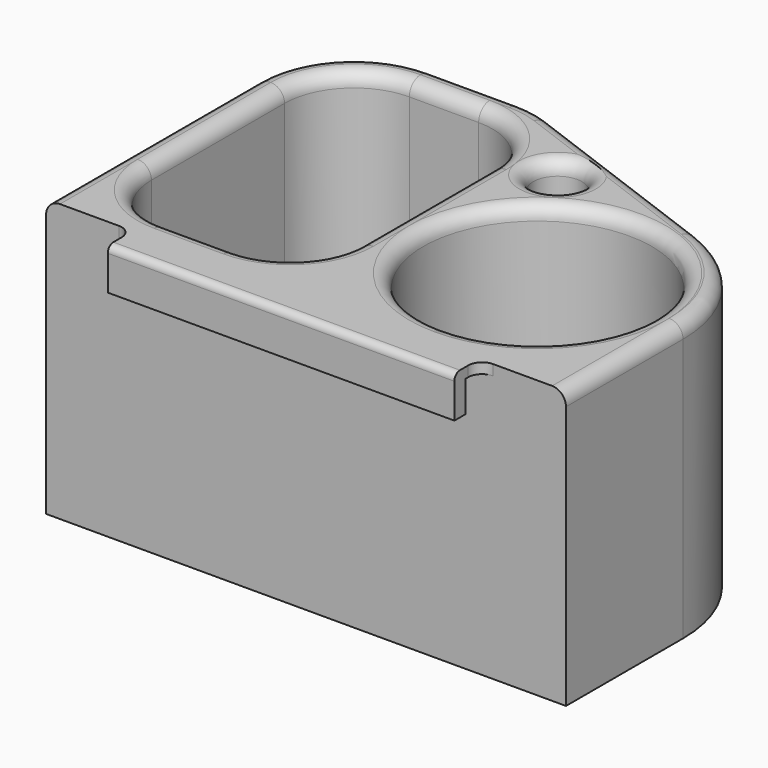
from build123d import *

# Parameters (mm, degrees)
F0_R         = 16.5
F0_R_2       = 3.5170103203
F1_DEPTH     = 40
F2_R         = 16.5
F3_DEPTH     = 38
F4_W         = 50
F4_H         = 34
F5_DEPTH     = 4.5
F6_W         = 50
F6_H         = 2.5
F7_DEPTH     = 4.5
F8_T1_DEPTH  = 1.5
F8_T3_DEPTH  = 24
F8_T5_DEPTH  = 32.3129968036
F8_T7_DEPTH  = 12.8102496977
F8_T9_DEPTH  = 43
F8_T11_DEPTH = 26.1042093904
F8_T13_DEPTH = 10
F8_T20_ANGLE = 69.5823366889
F8_T22_ANGLE = 20.4176633111
F8_T24_ANGLE = 90
F8_T26_ANGLE = 90
F8_T28_ANGLE = 90
F8_T30_ANGLE = 90
F8_T32_ANGLE = 90
F9_R         = 1


# Not quite as in the source:
# - a fillet or chamfer that OpenCascade refuses, or shapes differently, is made with other operations: its cross-section is extruded or revolved along the edge and cut away or added


with BuildPart() as f1:
    # F0 (on Top) → F1 (new body)
    with BuildSketch(Plane.XY):
        with BuildLine():
            Line((0, 38), (0, 0))
            Line((0, 0), (12.5, 0))
            Line((12.5, 0), (12.5, -4.5))
            Line((12.5, -4.5), (62.5, -4.5))
            Line((62.5, -4.5), (62.5, 0))
            Line((62.5, 0), (75, 0))
            Line((75, 0), (75, 21.1042093904))
            ThreePointArc((75, 21.1042093904), (71.4247434001, 32.5159491456), (61.9772195759, 39.8476991132))
            Line((61.9772195759, 39.8476991132), (31.6943034009, 51.120442806))
            ThreePointArc((31.6943034009, 51.120442806), (29.2915599077, 51.7783562025), (26.8102496977, 52))
            Line((26.8102496977, 52), (14, 52))
            ThreePointArc((14, 52), (4.1005050634, 47.8994949366), (0, 38))
        make_face()
        with Locations((54.5, 20.5)):
            Circle(F0_R, mode=Mode.SUBTRACT)
        with BuildLine():
            ThreePointArc((4, 38), (6.9289321881, 45.0710678119), (14, 48))
            Line((14, 48), (24, 48))
            ThreePointArc((24, 48), (31.0710678119, 45.0710678119), (34, 38))
            Line((34, 38), (34, 14))
            ThreePointArc((34, 14), (31.0710678119, 6.9289321881), (24, 4))
            Line((24, 4), (14, 4))
            ThreePointArc((14, 4), (6.9289321881, 6.9289321881), (4, 14))
            Line((4, 14), (4, 38))
        make_face(mode=Mode.SUBTRACT)
        with Locations((41.3257834749, 40.5812550323)):
            Circle(F0_R_2, mode=Mode.SUBTRACT)
        with Locations((54.5, 20.5)):
            Circle(F0_R)
    extrude(amount=F1_DEPTH)

    # F2 (on face) → F3 (cut)
    with BuildSketch(Plane.XY.offset(40)):
        with Locations((54.5, 20.5)):
            Circle(F2_R)
    extrude(amount=-F3_DEPTH, mode=Mode.SUBTRACT)

    # F4 (on face) → F5 (cut)
    with BuildSketch(Plane.XZ.offset(4.5)):
        with Locations((37.5, 17)):
            Rectangle(F4_W, F4_H)
    extrude(amount=-F5_DEPTH, mode=Mode.SUBTRACT)

    # F6 (on face) → F7 (cut)
    with BuildSketch(Plane(origin=(0, 0, 34), x_dir=(1, 0, 0), z_dir=(0, 0, -1))):
        with Locations((37.5, 1.25)):
            Rectangle(F6_W, F6_H)
    extrude(amount=-F7_DEPTH, mode=Mode.SUBTRACT)

    # F8: fillet of radius 2 on 6 edges, made by hand

    # F8_s2 → F8_t1 (join)
    with BuildSketch(Plane.XY.offset(38.5)):
        with BuildLine():
            ThreePointArc((10.5, 0), (11.9142135624, -0.5857864376), (12.5, -2))
            Line((12.5, -2), (12.5, 0))
            Line((12.5, 0), (10.5, 0))
        make_face()
        with BuildLine():
            ThreePointArc((64.5, 0), (63.0857864376, -0.5857864376), (62.5, -2))
            Line((62.5, -2), (62.5, 0))
            Line((62.5, 0), (64.5, 0))
        make_face()
    extrude(amount=F8_T1_DEPTH)

    # F8_s4 → F8_t3 (cut)
    with BuildSketch(Plane.XZ.offset(-38)):
        with BuildLine():
            ThreePointArc((36, 40), (34.5857864376, 39.4142135624), (34, 38))
            Line((34, 38), (34, 40))
            Line((34, 40), (36, 40))
        make_face()
        with BuildLine():
            ThreePointArc((2, 40), (3.4142135624, 39.4142135624), (4, 38))
            Line((4, 38), (4, 40))
            Line((4, 40), (2, 40))
        make_face()
    extrude(amount=F8_T3_DEPTH, mode=Mode.SUBTRACT)

    # F8_s6 → F8_t5 (cut)
    with BuildSketch(Plane(origin=(41.4063945876, -15.4134321387, 0), x_dir=(0, 0, 1), z_dir=(-0.9371744861, 0.3488609788, 0))):
        with BuildLine():
            ThreePointArc((40, 56.9656804247), (39.4142135624, 58.3798939871), (38, 58.9656804247))
            Line((38, 58.9656804247), (40, 58.9656804247))
            Line((40, 58.9656804247), (40, 56.9656804247))
        make_face()
    extrude(amount=F8_T5_DEPTH, mode=Mode.SUBTRACT)

    # F8_s8 → F8_t7 (cut)
    with BuildSketch(Plane.YZ.offset(14)):
        with BuildLine():
            ThreePointArc((50, 40), (51.4142135624, 39.4142135624), (52, 38))
            Line((52, 38), (52, 40))
            Line((52, 40), (50, 40))
        make_face()
    extrude(amount=F8_T7_DEPTH, mode=Mode.SUBTRACT)

    # F8_s10 → F8_t9 (cut)
    with BuildSketch(Plane.XZ.offset(-38)):
        with BuildLine():
            ThreePointArc((2, 40), (0.5857864376, 39.4142135624), (0, 38))
            Line((0, 38), (0, 40))
            Line((0, 40), (2, 40))
        make_face()
    extrude(amount=F8_T9_DEPTH, mode=Mode.SUBTRACT)

    # F8_s12 → F8_t11 (cut)
    with BuildSketch(Plane.XZ.offset(-21.1042093904)):
        with BuildLine():
            ThreePointArc((73, 40), (74.4142135624, 39.4142135624), (75, 38))
            Line((75, 38), (75, 40))
            Line((75, 40), (73, 40))
        make_face()
    extrude(amount=F8_T11_DEPTH, mode=Mode.SUBTRACT)

    # F8_s14 → F8_t13 (cut)
    with BuildSketch(Plane.YZ.offset(14)):
        with BuildLine():
            ThreePointArc((2, 40), (3.4142135624, 39.4142135624), (4, 38))
            Line((4, 38), (4, 40))
            Line((4, 40), (2, 40))
        make_face()
        with BuildLine():
            ThreePointArc((50, 40), (48.5857864376, 39.4142135624), (48, 38))
            Line((48, 38), (48, 40))
            Line((48, 40), (50, 40))
        make_face()
    extrude(amount=F8_T13_DEPTH, mode=Mode.SUBTRACT)

    # F8_s15 → F8_t16 (revolve, cut)
    with BuildSketch(Plane.XZ.offset(-20.5)):
        with BuildLine():
            ThreePointArc((73, 40), (71.5857864376, 39.4142135624), (71, 38))
            Line((71, 38), (71, 40))
            Line((71, 40), (73, 40))
        make_face()
    revolve(axis=Axis((54.5, 20.5, 40), (0, 0, 1)), mode=Mode.SUBTRACT)

    # F8_s17 → F8_t18 (revolve, cut)
    with BuildSketch(Plane.XZ.offset(-40.5812550323)):
        with BuildLine():
            ThreePointArc((46.8427937951, 40), (45.4285802328, 39.4142135624), (44.8427937951, 38))
            Line((44.8427937951, 38), (44.8427937951, 40))
            Line((44.8427937951, 40), (46.8427937951, 40))
        make_face()
    revolve(axis=Axis((41.3257834749, 40.5812550323, 40), (0, 0, 1)), mode=Mode.SUBTRACT)

    # F8_s19 → F8_t20 (revolve, cut)
    with BuildSketch(Plane.XZ.offset(-21.1042093904)):
        with BuildLine():
            ThreePointArc((73, 40), (74.4142135624, 39.4142135624), (75, 38))
            Line((75, 38), (75, 40))
            Line((75, 40), (73, 40))
        make_face()
    revolve(axis=Axis((55, 21.1042093904, 40), (0, 0, 1)), revolution_arc=F8_T20_ANGLE, mode=Mode.SUBTRACT)

    # F8_s21 → F8_t22 (revolve, cut)
    with BuildSketch(Plane(origin=(11.1234784125, -4.140688446, 0), x_dir=(0, 0, 1), z_dir=(0.9371744861, -0.3488609788, 0))):
        with BuildLine():
            ThreePointArc((38, -58.9656804247), (39.4142135624, -58.3798939871), (40, -56.9656804247))
            Line((40, -56.9656804247), (40, -58.9656804247))
            Line((40, -58.9656804247), (38, -58.9656804247))
        make_face()
    revolve(axis=Axis((26.8102496977, 38, 40), (0, 0, 1)), revolution_arc=F8_T22_ANGLE, mode=Mode.SUBTRACT)

    # F8_s23 → F8_t24 (revolve, cut)
    with BuildSketch(Plane.YZ.offset(14)):
        with BuildLine():
            ThreePointArc((50, 40), (51.4142135624, 39.4142135624), (52, 38))
            Line((52, 38), (52, 40))
            Line((52, 40), (50, 40))
        make_face()
    revolve(axis=Axis((14, 38, 40), (0, 0, 1)), revolution_arc=F8_T24_ANGLE, mode=Mode.SUBTRACT)

    # F8_s25 → F8_t26 (revolve, cut)
    with BuildSketch(Plane.YZ.offset(24)):
        with BuildLine():
            ThreePointArc((50, 40), (48.5857864376, 39.4142135624), (48, 38))
            Line((48, 38), (48, 40))
            Line((48, 40), (50, 40))
        make_face()
    revolve(axis=Axis((24, 38, 40), (0, 0, -1)), revolution_arc=F8_T26_ANGLE, mode=Mode.SUBTRACT)

    # F8_s27 → F8_t28 (revolve, cut)
    with BuildSketch(Plane.XZ.offset(-14)):
        with BuildLine():
            ThreePointArc((36, 40), (34.5857864376, 39.4142135624), (34, 38))
            Line((34, 38), (34, 40))
            Line((34, 40), (36, 40))
        make_face()
    revolve(axis=Axis((24, 14, 40), (0, 0, -1)), revolution_arc=F8_T28_ANGLE, mode=Mode.SUBTRACT)

    # F8_s29 → F8_t30 (revolve, cut)
    with BuildSketch(Plane.YZ.offset(14)):
        with BuildLine():
            ThreePointArc((2, 40), (3.4142135624, 39.4142135624), (4, 38))
            Line((4, 38), (4, 40))
            Line((4, 40), (2, 40))
        make_face()
    revolve(axis=Axis((14, 14, 40), (0, 0, -1)), revolution_arc=F8_T30_ANGLE, mode=Mode.SUBTRACT)

    # F8_s31 → F8_t32 (revolve, cut)
    with BuildSketch(Plane.XZ.offset(-38)):
        with BuildLine():
            ThreePointArc((2, 40), (3.4142135624, 39.4142135624), (4, 38))
            Line((4, 38), (4, 40))
            Line((4, 40), (2, 40))
        make_face()
    revolve(axis=Axis((14, 38, 40), (0, 0, -1)), revolution_arc=F8_T32_ANGLE, mode=Mode.SUBTRACT)

    # F9
    f9_edges = [f1.edges().sort_by_distance(p)[0] for p in [
        (37.5, -4.5, 40),
    ]]
    fillet(f9_edges, radius=F9_R)


solid = f1.part
